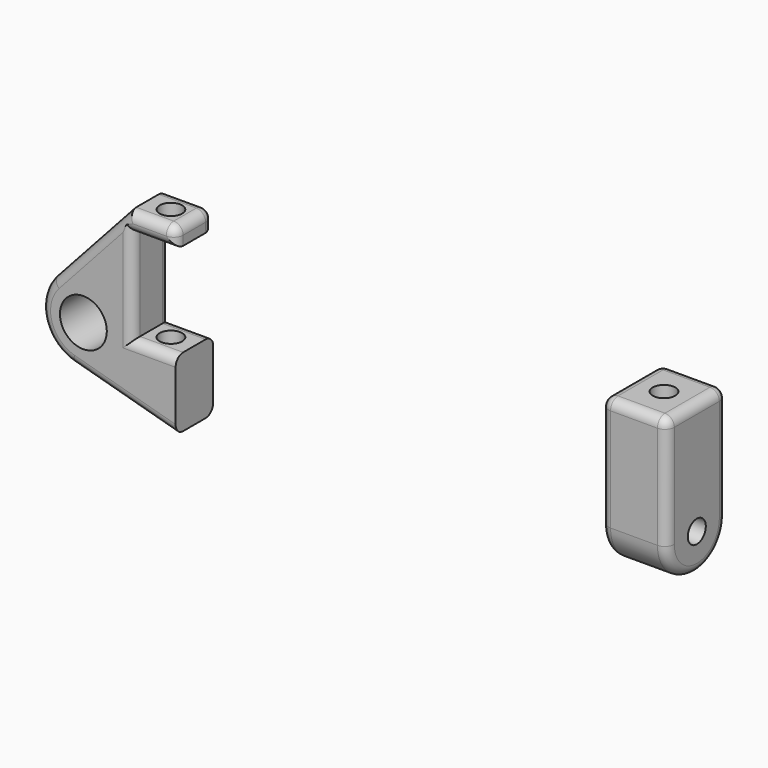
from build123d import *

# Parameters (mm, degrees)
F0_R          = 3.175
F2_DEPTH      = 3.175
F3_R          = 1.524
F4_DEPTH      = 7.62
F4_DEPTH_BACK = 1.27
F5_DEPTH      = 56.134
F7_R          = 1.524
F8_DEPTH      = 17.78
F6_R          = 1.524
F9_DEPTH      = 10.414
F10_T1_DEPTH  = 18.5821257943
F10_T3_DEPTH  = 8.255
F10_T5_DEPTH  = 4.445
F10_T7_DEPTH  = 9.017
F10_T9_DEPTH  = 12.7
F10_T11_DEPTH = 17.7294216388
F10_T13_DEPTH = 3.81
F10_S17_W     = 1.27
F10_S17_H     = 1.27
F10_T18_DEPTH = 1.27
F10_S23_W     = 1.27
F10_S23_H     = 1.27
F10_T24_DEPTH = 1.27
F10_T28_ANGLE = 116.8111069241
F10_T30_ANGLE = 116.8111069241
F10_T35_DEPTH = 15.875
F10_T39_DEPTH = 12.192
F10_T46_DEPTH = 15.875
F10_T50_DEPTH = 12.192
F10_T57_DEPTH = 15.875
F10_T61_DEPTH = 12.192
F10_T68_DEPTH = 15.875
F10_T72_DEPTH = 12.192
F10_2_F1_R    = 1.27
F10_2_F2_R    = 1.27
F10_2_F3_R    = 1.27


# Not quite as in the source:
# - a fillet or chamfer that OpenCascade refuses, or shapes differently, is made with other operations: its cross-section is extruded or revolved along the edge and cut away or added
# - two fillets or chamfers of one size are made in one step
# - the program builds the solid bodies; features that only make, move or delete a surface that nothing else refers to are left out


with BuildPart() as f2:
    # F0 (on Front) → F2 (new body, symmetric)
    with BuildSketch(Plane.XZ):
        with BuildLine():
            Line((-0.9398, 0), (0, 0))
            Line((0, 0), (0, 12.7))
            Line((0, 12.7), (5.842, 12.7))
            Line((5.842, 12.7), (5.842, 15.24))
            Line((5.842, 15.24), (-0.508, 15.24))
            Line((-0.508, 15.24), (-10.8806298187, 3.8475430269))
            ThreePointArc((-10.8806298187, 3.8475430269), (-4.5919612295, 5.3297205562), (-0.9398, 0))
        make_face()
        with BuildLine():
            ThreePointArc((-8.1826630726, -5.5069827884), (-3.1957909266, -4.5493385486), (-0.9398, 0))
            ThreePointArc((-0.9398, 0), (-4.5919612295, 5.3297205562), (-10.8806298187, 3.8475430269))
            ThreePointArc((-10.8806298187, 3.8475430269), (-12.1459778134, -1.5837270034), (-8.1826630726, -5.5069827884))
        make_face()
        with Locations((-6.6548, 0)):
            Circle(F0_R, mode=Mode.SUBTRACT)
        with BuildLine():
            Line((5.842, 0), (0, 0))
            Line((0, 0), (-0.9398, 0))
            ThreePointArc((-0.9398, 0), (-3.1957909266, -4.5493385486), (-8.1826630726, -5.5069827884))
            Line((-8.1826630726, -5.5069827884), (5.842, -9.398))
            Line((5.842, -9.398), (5.842, 0))
        make_face()
    extrude(amount=F2_DEPTH, both=True)

    # F3 (on face) → F5 (cut)
    with BuildSketch(Plane.YZ.offset(66.294)):
        Circle(F3_R)
    extrude(amount=-F5_DEPTH, mode=Mode.SUBTRACT)

    # F7 (on face) → F8 (cut)
    with BuildSketch(Plane.XY.offset(15.24)):
        with Locations((2.667, 0)):
            Circle(F7_R)
    extrude(amount=-F8_DEPTH, mode=Mode.SUBTRACT)

    # F10: fillet of radius 1.27 on 17 edges, made by hand

    # F10_s2 → F10_t1 (cut)
    with BuildSketch(Plane(origin=(9.4938886236, 0, 10.4273187748), x_dir=(0, 1, 0), z_dir=(-0.6732358752, 0, -0.7394277898))):
        with BuildLine():
            ThreePointArc((-3.175, -9.3657440555), (-2.8030256121, -10.2637696676), (-1.905, -10.6357440555))
            Line((-1.905, -10.6357440555), (-3.175, -10.6357440555))
            Line((-3.175, -10.6357440555), (-3.175, -9.3657440555))
        make_face()
        with BuildLine():
            ThreePointArc((3.175, -9.3657440555), (2.8030256121, -10.2637696676), (1.905, -10.6357440555))
            Line((1.905, -10.6357440555), (3.175, -10.6357440555))
            Line((3.175, -10.6357440555), (3.175, -9.3657440555))
        make_face()
    extrude(amount=F10_T1_DEPTH, mode=Mode.SUBTRACT)

    # F10_s4 → F10_t3 (cut)
    with BuildSketch(Plane.YZ.offset(-3.683)):
        with BuildLine():
            ThreePointArc((-3.175, 13.97), (-2.8030256121, 14.8680256121), (-1.905, 15.24))
            Line((-1.905, 15.24), (-3.175, 15.24))
            Line((-3.175, 15.24), (-3.175, 13.97))
        make_face()
        with BuildLine():
            ThreePointArc((3.175, 13.97), (2.8030256121, 14.8680256121), (1.905, 15.24))
            Line((1.905, 15.24), (3.175, 15.24))
            Line((3.175, 15.24), (3.175, 13.97))
        make_face()
    extrude(amount=F10_T3_DEPTH, mode=Mode.SUBTRACT)

    # F10_s6 → F10_t5 (cut)
    with BuildSketch(Plane.XY.offset(9.525)):
        with BuildLine():
            ThreePointArc((4.572, -3.175), (5.4700256121, -2.8030256121), (5.842, -1.905))
            Line((5.842, -1.905), (5.842, -3.175))
            Line((5.842, -3.175), (4.572, -3.175))
        make_face()
        with BuildLine():
            ThreePointArc((4.572, 3.175), (5.4700256121, 2.8030256121), (5.842, 1.905))
            Line((5.842, 1.905), (5.842, 3.175))
            Line((5.842, 3.175), (4.572, 3.175))
        make_face()
    extrude(amount=F10_T5_DEPTH, mode=Mode.SUBTRACT)

    # F10_s8 → F10_t7 (cut)
    with BuildSketch(Plane.YZ):
        with BuildLine():
            ThreePointArc((-1.905, 12.7), (-2.8030256121, 13.0719743879), (-3.175, 13.97))
            Line((-3.175, 13.97), (-3.175, 12.7))
            Line((-3.175, 12.7), (-1.905, 12.7))
        make_face()
        with BuildLine():
            ThreePointArc((3.175, 13.97), (2.8030256121, 13.0719743879), (1.905, 12.7))
            Line((1.905, 12.7), (3.175, 12.7))
            Line((3.175, 12.7), (3.175, 13.97))
        make_face()
        with BuildLine():
            ThreePointArc((3.175, -1.27), (2.8030256121, -0.3719743879), (1.905, 0))
            Line((1.905, 0), (3.175, 0))
            Line((3.175, 0), (3.175, -1.27))
        make_face()
        with BuildLine():
            ThreePointArc((-3.175, -1.27), (-2.8030256121, -0.3719743879), (-1.905, 0))
            Line((-1.905, 0), (-3.175, 0))
            Line((-3.175, 0), (-3.175, -1.27))
        make_face()
    extrude(amount=F10_T7_DEPTH, mode=Mode.SUBTRACT)

    # F10_s10 → F10_t9 (cut)
    with BuildSketch(Plane.XY):
        with BuildLine():
            ThreePointArc((0, -1.905), (-0.3719743879, -2.8030256121), (-1.27, -3.175))
            Line((-1.27, -3.175), (0, -3.175))
            Line((0, -3.175), (0, -1.905))
        make_face()
        with BuildLine():
            ThreePointArc((0, 1.905), (-0.3719743879, 2.8030256121), (-1.27, 3.175))
            Line((-1.27, 3.175), (0, 3.175))
            Line((0, 3.175), (0, 1.905))
        make_face()
    extrude(amount=F10_T9_DEPTH, mode=Mode.SUBTRACT)

    # F10_s12 → F10_t11 (cut)
    with BuildSketch(Plane(origin=(-6.179167626, 0, 1.7143547379), x_dir=(0, 1, 0), z_dir=(0.9636015378, 0, -0.2673426199))):
        with BuildLine():
            ThreePointArc((-3.175, -6.2241116667), (-2.8030256121, -7.1221372788), (-1.905, -7.4941116667))
            Line((-1.905, -7.4941116667), (-3.175, -7.4941116667))
            Line((-3.175, -7.4941116667), (-3.175, -6.2241116667))
        make_face()
        with BuildLine():
            ThreePointArc((3.175, -6.2241116667), (2.8030256121, -7.1221372788), (1.905, -7.4941116667))
            Line((1.905, -7.4941116667), (3.175, -7.4941116667))
            Line((3.175, -7.4941116667), (3.175, -6.2241116667))
        make_face()
    extrude(amount=F10_T11_DEPTH, mode=Mode.SUBTRACT)

    # F10_s14 → F10_t13 (cut)
    with BuildSketch(Plane.XZ.offset(-1.905)):
        with BuildLine():
            ThreePointArc((5.842, 13.97), (5.4700256121, 14.8680256121), (4.572, 15.24))
            Line((4.572, 15.24), (5.842, 15.24))
            Line((5.842, 15.24), (5.842, 13.97))
        make_face()
    extrude(amount=F10_T13_DEPTH, mode=Mode.SUBTRACT)


with BuildPart() as f4:
    # F3 (on face) → F4 (new body, two sides)
    with BuildSketch(Plane.YZ.offset(66.294)) as f4_sk:
        with BuildLine():
            ThreePointArc((-5.08, 0), (0, -5.08), (5.08, 0))
            ThreePointArc((5.08, 0), (0, 5.08), (-5.08, 0))
        make_face()
        Circle(F3_R, mode=Mode.SUBTRACT)
        with BuildLine():
            ThreePointArc((-5.08, 0), (0, 5.08), (5.08, 0))
            Line((5.08, 0), (5.08, 15.24))
            Line((5.08, 15.24), (-5.08, 15.24))
            Line((-5.08, 15.24), (-5.08, 0))
        make_face()
    extrude(amount=F4_DEPTH)
    extrude(f4_sk.sketch, amount=-F4_DEPTH_BACK)

    # F6 (on face) → F9 (cut)
    with BuildSketch(Plane.XY.offset(15.24)):
        with Locations((69.469, 0)):
            Circle(F6_R)
    extrude(amount=-F9_DEPTH, mode=Mode.SUBTRACT)

    # F10#2: fillet of radius 1.27 on 10 edges, made by hand

    # F10_2_f1
    f10_2_f1_edges = [f4.edges().sort_by_distance(p)[0] for p in [
        (73.914, 0, -5.08),
        (73.914, -5.08, 7.62),
        (73.914, 5.08, 7.62),
    ]]
    fillet(f10_2_f1_edges, radius=F10_2_F1_R)

    # F10_2_f2
    f10_2_f2_edges = [f4.edges().sort_by_distance(p)[0] for p in [
        (65.024, 0, -5.08),
        (65.024, -5.08, 7.62),
        (65.024, 5.08, 7.62),
    ]]
    fillet(f10_2_f2_edges, radius=F10_2_F2_R)

    # F10_2_f3
    f10_2_f3_edges = [f4.edges().sort_by_distance(p)[0] for p in [
        (69.469, -5.08, 15.24),
    ]]
    fillet(f10_2_f3_edges, radius=F10_2_F3_R)


with BuildPart() as f10_tool16:
    # F10_s17 → F10_t18 (new body)
    with BuildSketch(Plane.XZ.offset(1.905)):
        with Locations((5.207, 14.605)):
            Rectangle(F10_S17_W, F10_S17_H)
    extrude(amount=F10_T18_DEPTH)

    # F10_s19 → F10_t20 (revolve, cut)
    with BuildSketch(Plane(origin=(4.572, -1.905, 13.97), x_dir=(-0.7071067812, 0, -0.7071067812), z_dir=(-0.7071067812, 0, 0.7071067812))):
        with BuildLine():
            ThreePointArc((0, -1.27), (1.27, 0), (0, 1.27))
            Line((0, 1.27), (0, -1.27))
        make_face()
    revolve(axis=Axis((4.572, -1.905, 13.97), (0, -1, 0)), mode=Mode.SUBTRACT)


with BuildPart() as f2_1:
    add(f2.part)

    # F10_t15: cut F10_tool16
    add(f10_tool16.part, mode=Mode.SUBTRACT)


with BuildPart() as f10_tool22:
    # F10_s23 → F10_t24 (new body)
    with BuildSketch(Plane.XZ.offset(-1.905)):
        with Locations((5.207, 14.605)):
            Rectangle(F10_S23_W, F10_S23_H)
    extrude(amount=-F10_T24_DEPTH)

    # F10_s25 → F10_t26 (revolve, cut)
    with BuildSketch(Plane(origin=(4.572, 1.905, 13.97), x_dir=(-0.7071067812, 0, -0.7071067812), z_dir=(0.7071067812, 0, -0.7071067812))):
        with BuildLine():
            ThreePointArc((0, -1.27), (1.27, 0), (0, 1.27))
            Line((0, 1.27), (0, -1.27))
        make_face()
    revolve(axis=Axis((4.572, 1.905, 13.97), (0, 1, 0)), mode=Mode.SUBTRACT)


with BuildPart() as f2_2:
    add(f2_1.part)

    # F10_t21: cut F10_tool22
    add(f10_tool22.part, mode=Mode.SUBTRACT)

    # F10_s27 → F10_t28 (revolve, cut)
    with BuildSketch(Plane(origin=(-3.0162650989, 0, -3.3128214309), x_dir=(0, 1, 0), z_dir=(0.6732358752, 0, 0.7394277898))):
        with BuildLine():
            ThreePointArc((-3.175, 9.3657440555), (-2.8030256121, 10.2637696676), (-1.905, 10.6357440555))
            Line((-1.905, 10.6357440555), (-3.175, 10.6357440555))
            Line((-3.175, 10.6357440555), (-3.175, 9.3657440555))
        make_face()
    revolve(axis=Axis((-6.6548, -3.175, 0), (0, -1, 0)), revolution_arc=F10_T28_ANGLE, mode=Mode.SUBTRACT)

    # F10_s29 → F10_t30 (revolve, cut)
    with BuildSketch(Plane(origin=(-3.0162650989, 0, -3.3128214309), x_dir=(0, 1, 0), z_dir=(0.6732358752, 0, 0.7394277898))):
        with BuildLine():
            ThreePointArc((3.175, 9.3657440555), (2.8030256121, 10.2637696676), (1.905, 10.6357440555))
            Line((1.905, 10.6357440555), (3.175, 10.6357440555))
            Line((3.175, 10.6357440555), (3.175, 9.3657440555))
        make_face()
    revolve(axis=Axis((-6.6548, 3.175, 0), (0, -1, 0)), revolution_arc=F10_T30_ANGLE, mode=Mode.SUBTRACT)


with BuildPart() as f10_tool33:
    # F10_s34 → F10_t35 (new body)
    with BuildSketch(Plane.XY):
        with BuildLine():
            ThreePointArc((0, -1.905), (-0.3719743879, -2.8030256121), (-1.27, -3.175))
            Line((-1.27, -3.175), (0, -3.175))
            Line((0, -3.175), (0, -1.905))
        make_face()
    extrude(amount=F10_T35_DEPTH)

    split(bisect_by=Plane.XY.offset(12.7), keep=Keep.TOP)


with BuildPart() as f10_tool37:
    # F10_s38 → F10_t39 (new body)
    with BuildSketch(Plane.YZ.offset(-3.175)):
        with BuildLine():
            ThreePointArc((-1.905, 12.7), (-2.8030256121, 13.0719743879), (-3.175, 13.97))
            Line((-3.175, 13.97), (-3.175, 12.7))
            Line((-3.175, 12.7), (-1.905, 12.7))
        make_face()
    extrude(amount=F10_T39_DEPTH)

    split(bisect_by=Plane.YZ, keep=Keep.BOTTOM)


with BuildPart() as f10_tool33_1:
    add(f10_tool33.part)

    # F10_t41: intersect F10_tool37
    add(f10_tool37.part, mode=Mode.INTERSECT)


with BuildPart() as f2_3:
    add(f2_2.part)

    # F10_t31: cut F10_tool33
    add(f10_tool33_1.part, mode=Mode.SUBTRACT)


with BuildPart() as f10_tool44:
    # F10_s45 → F10_t46 (new body)
    with BuildSketch(Plane.XY.offset(-3.175)):
        with BuildLine():
            ThreePointArc((0, -1.905), (-0.3719743879, -2.8030256121), (-1.27, -3.175))
            Line((-1.27, -3.175), (0, -3.175))
            Line((0, -3.175), (0, -1.905))
        make_face()
    extrude(amount=F10_T46_DEPTH)

    split(bisect_by=Plane.XY, keep=Keep.BOTTOM)


with BuildPart() as f10_tool48:
    # F10_s49 → F10_t50 (new body)
    with BuildSketch(Plane.YZ.offset(9.017)):
        with BuildLine():
            ThreePointArc((-3.175, -1.27), (-2.8030256121, -0.3719743879), (-1.905, 0))
            Line((-1.905, 0), (-3.175, 0))
            Line((-3.175, 0), (-3.175, -1.27))
        make_face()
    extrude(amount=-F10_T50_DEPTH)

    split(bisect_by=Plane.YZ, keep=Keep.BOTTOM)


with BuildPart() as f10_tool44_1:
    add(f10_tool44.part)

    # F10_t52: intersect F10_tool48
    add(f10_tool48.part, mode=Mode.INTERSECT)


with BuildPart() as f2_4:
    add(f2_3.part)

    # F10_t42: cut F10_tool44
    add(f10_tool44_1.part, mode=Mode.SUBTRACT)


with BuildPart() as f10_tool55:
    # F10_s56 → F10_t57 (new body)
    with BuildSketch(Plane.XY):
        with BuildLine():
            ThreePointArc((0, 1.905), (-0.3719743879, 2.8030256121), (-1.27, 3.175))
            Line((-1.27, 3.175), (0, 3.175))
            Line((0, 3.175), (0, 1.905))
        make_face()
    extrude(amount=F10_T57_DEPTH)

    split(bisect_by=Plane.XY.offset(12.7), keep=Keep.TOP)


with BuildPart() as f10_tool59:
    # F10_s60 → F10_t61 (new body)
    with BuildSketch(Plane.YZ.offset(-3.175)):
        with BuildLine():
            ThreePointArc((3.175, 13.97), (2.8030256121, 13.0719743879), (1.905, 12.7))
            Line((1.905, 12.7), (3.175, 12.7))
            Line((3.175, 12.7), (3.175, 13.97))
        make_face()
    extrude(amount=F10_T61_DEPTH)

    split(bisect_by=Plane.YZ, keep=Keep.BOTTOM)


with BuildPart() as f10_tool55_1:
    add(f10_tool55.part)

    # F10_t63: intersect F10_tool59
    add(f10_tool59.part, mode=Mode.INTERSECT)


with BuildPart() as f2_5:
    add(f2_4.part)

    # F10_t53: cut F10_tool55
    add(f10_tool55_1.part, mode=Mode.SUBTRACT)


with BuildPart() as f10_tool66:
    # F10_s67 → F10_t68 (new body)
    with BuildSketch(Plane.XY.offset(-3.175)):
        with BuildLine():
            ThreePointArc((0, 1.905), (-0.3719743879, 2.8030256121), (-1.27, 3.175))
            Line((-1.27, 3.175), (0, 3.175))
            Line((0, 3.175), (0, 1.905))
        make_face()
    extrude(amount=F10_T68_DEPTH)

    split(bisect_by=Plane.XY, keep=Keep.BOTTOM)


with BuildPart() as f10_tool70:
    # F10_s71 → F10_t72 (new body)
    with BuildSketch(Plane.YZ.offset(9.017)):
        with BuildLine():
            ThreePointArc((3.175, -1.27), (2.8030256121, -0.3719743879), (1.905, 0))
            Line((1.905, 0), (3.175, 0))
            Line((3.175, 0), (3.175, -1.27))
        make_face()
    extrude(amount=-F10_T72_DEPTH)

    split(bisect_by=Plane.YZ, keep=Keep.BOTTOM)


with BuildPart() as f10_tool66_1:
    add(f10_tool66.part)

    # F10_t74: intersect F10_tool70
    add(f10_tool70.part, mode=Mode.INTERSECT)


with BuildPart() as f2_6:
    add(f2_5.part)

    # F10_t64: cut F10_tool66
    add(f10_tool66_1.part, mode=Mode.SUBTRACT)


solid = Compound([f4.part, f2_6.part])
